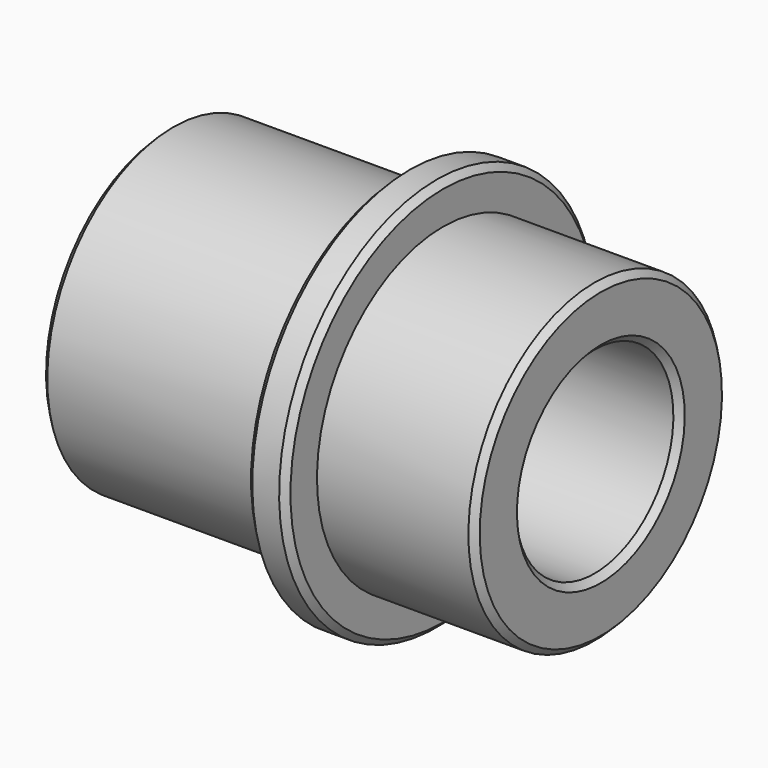
from build123d import *


# Not quite as in the source:
# - a fillet or chamfer that OpenCascade refuses, or shapes differently, is made with other operations: its cross-section is extruded or revolved along the edge and cut away or added


with BuildPart() as f1:
    # F0 (on Front) → F1 (revolve)
    with BuildSketch(Plane.XZ):
        Polygon((-22.5108576886, 12.7), (-41.5608576886, 12.7), (-41.5608576886, 9.525), (-22.5108576886, 7.9375), (-6.6358576886, 7.9375), (-6.6358576886, 12.7), (-19.3358576886, 12.7), (-19.3358576886, 15.875), (-22.5108576886, 15.875), align=None)
    revolve(axis=Axis((-22.7388739586, 0, 0), (-1, 0, 0)))

    # F2: chamfer of 0.508 on 6 edges, made by hand

    # F2_s1 → F2_t2 (revolve, cut)
    with BuildSketch(Plane.XZ):
        Polygon((-22.0028576886, 15.875), (-22.5108576886, 15.367), (-22.5108576886, 15.875), align=None)
    revolve(axis=Axis((-22.5108576886, 0, 0), (-1, 0, 0)), mode=Mode.SUBTRACT)

    # F2_s3 → F2_t4 (revolve, cut)
    with BuildSketch(Plane.XZ):
        Polygon((-19.3358576886, 15.367), (-19.8438576886, 15.875), (-19.3358576886, 15.875), align=None)
    revolve(axis=Axis((-19.3358576886, 0, 0), (-1, 0, 0)), mode=Mode.SUBTRACT)

    # F2_s5 → F2_t6 (revolve, cut)
    with BuildSketch(Plane.XZ):
        Polygon((-41.0528576886, 12.7), (-41.5608576886, 12.192), (-41.5608576886, 12.7), align=None)
    revolve(axis=Axis((-41.5608576886, 0, 0), (-1, 0, 0)), mode=Mode.SUBTRACT)

    # F2_s7 → F2_t8 (revolve, cut)
    with BuildSketch(Plane.XZ):
        Polygon((-6.6358576886, 12.192), (-7.1438576886, 12.7), (-6.6358576886, 12.7), align=None)
    revolve(axis=Axis((-6.6358576886, 0, 0), (-1, 0, 0)), mode=Mode.SUBTRACT)

    # F2_s9 → F2_t10 (revolve, cut)
    with BuildSketch(Plane.XZ):
        Polygon((-41.5608576886, 9.9924275038), (-41.0950447924, 9.4861822586), (-41.5608576886, 9.525), align=None)
    revolve(axis=Axis((-41.5608576886, 0, 0), (-1, 0, 0)), mode=Mode.SUBTRACT)

    # F2_s11 → F2_t12 (revolve, cut)
    with BuildSketch(Plane.XZ):
        Polygon((-7.1438576886, 7.9375), (-6.6358576886, 8.4455), (-6.6358576886, 7.9375), align=None)
    revolve(axis=Axis((-6.6358576886, 0, 0), (-1, 0, 0)), mode=Mode.SUBTRACT)


solid = f1.part
